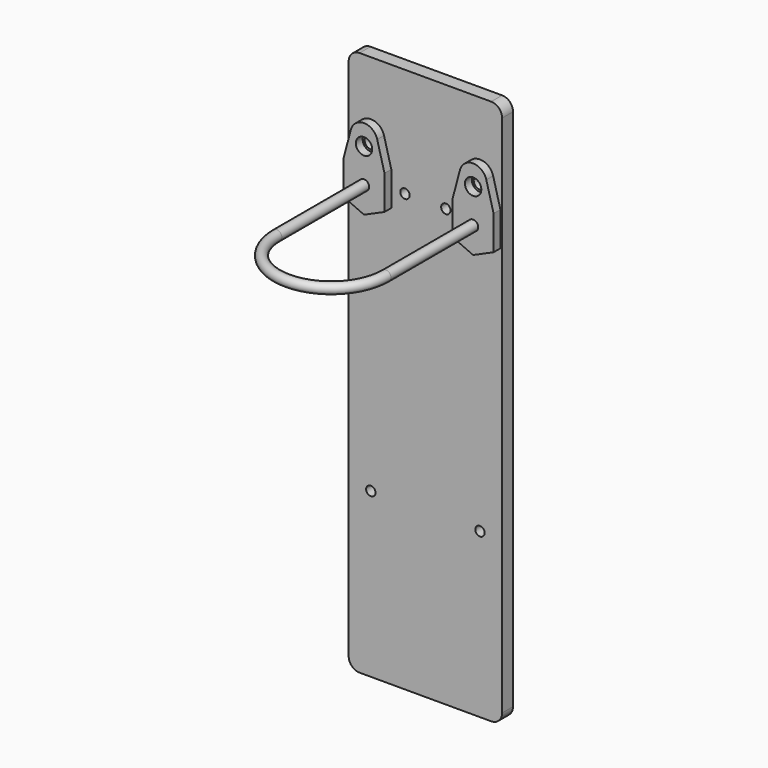
from build123d import *

# Parameters (mm, degrees)
F0_R     = 2.38125
F3_R     = 3.81
F4_DEPTH = 3.96875
F5_W     = 71.4375
F5_H     = 254
F5_R     = 2.1844
F5_R_2   = 2.8956
F6_DEPTH = 6.35
F7_R     = 5.08


# Not quite as in the source:
# - a pattern or mirror of a feature is missing from the dataset's text; its kind, count and spacing are read off the source's solid


with BuildPart() as f2:
    # F2: sweep along a path in F1
    with BuildLine(Plane.XY) as f2_path:
        Line((-25.4, 0), (-25.4, -50.8))
        ThreePointArc((-25.4, -50.8), (0, -76.2), (25.4, -50.8))
        Line((25.4, -50.8), (25.4, 0))
    # F0 (on Front) → F2 (sweep)
    with BuildSketch(Plane.XZ):
        with Locations((-25.4, 0)):
            Circle(F0_R)
    sweep(path=f2_path.line)

    # F3 (on Front) → F4 (join)
    with BuildSketch(Plane.XZ):
        with BuildLine():
            Line((34.925, 7.9375), (31.5368168318, 20.6815572844))
            ThreePointArc((31.5368168318, 20.6815572844), (25.4, 25.4), (19.2631831682, 20.6815572844))
            Line((19.2631831682, 20.6815572844), (15.875, 7.9375))
            Line((15.875, 7.9375), (15.875, -7.9375))
            Line((15.875, -7.9375), (25.4, -12.1708333333))
            Line((25.4, -12.1708333333), (34.925, -7.9375))
            Line((34.925, -7.9375), (34.925, 7.9375))
        make_face()
        with Locations((25.4, 15.875)):
            Circle(F3_R, mode=Mode.SUBTRACT)
    f4 = extrude(amount=-F4_DEPTH)

    # F4_copies: F4 across plane
    add(f4.mirror(Plane(origin=(0, 0, 0), x_dir=(0, 0, -1), z_dir=(-1, 0, 0))))


with BuildPart() as f6:
    # F5 (on face) → F6 (new body)
    with BuildSketch(Plane(origin=(0, 3.96875, 0), x_dir=(-1, 0, 0), z_dir=(0, 1, 0))):
        with Locations((0, -76.2)):
            Rectangle(F5_W, F5_H)
        with Locations((-25.4, -127)):
            Circle(F5_R, mode=Mode.SUBTRACT)
        with Locations((25.4, -127)):
            Circle(F5_R, mode=Mode.SUBTRACT)
        with Locations((-25.4, 15.875)):
            Circle(F5_R_2, mode=Mode.SUBTRACT)
        with Locations((-9.525, 0)):
            Circle(F5_R, mode=Mode.SUBTRACT)
        with Locations((9.525, 0)):
            Circle(F5_R, mode=Mode.SUBTRACT)
        with Locations((25.4, 15.875)):
            Circle(F5_R_2, mode=Mode.SUBTRACT)
    extrude(amount=F6_DEPTH)

    # F7
    f7_edges = [f6.edges().sort_by_distance(p)[0] for p in [
        (-35.71875, 7.14375, 50.8),
        (35.71875, 7.14375, 50.8),
        (35.71875, 7.14375, -203.2),
        (-35.71875, 7.14375, -203.2),
    ]]
    fillet(f7_edges, radius=F7_R)


solid = Compound([f2.part, f6.part])
